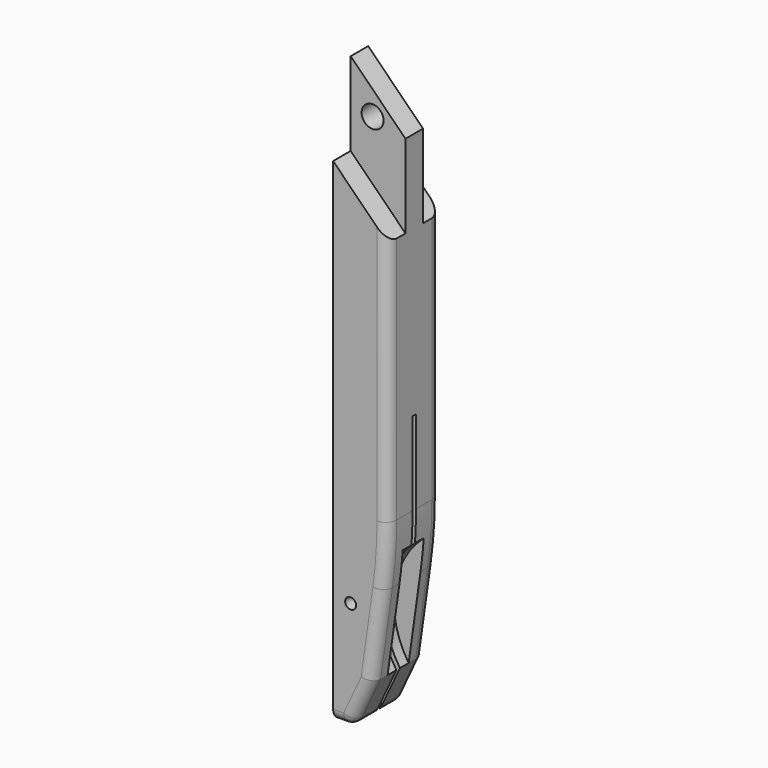
from build123d import *

# Parameters (mm, degrees)
F0_R      = 0.635
F1_DEPTH  = 3.81
F2_R      = 0.635
F3_DEPTH  = 0.254
F5_DEPTH  = 1.524
F7_DEPTH  = 1.524
F9_R      = 1.016
F10_DEPTH = 6.604
F0_R_2    = 1.27
F11_DEPTH = 1.27
F12_R     = 1.27


# Not quite as in the source:
# - two fillets or chamfers of one size are made in one step
# - a pattern or mirror of a feature is missing from the dataset's text; its kind, count and spacing are read off the source's solid


with BuildPart() as f1:
    # F0 (on Front) → F1 (new body)
    with BuildSketch(Plane.XZ):
        with BuildLine():
            Line((6.35, 50.8), (0, 57.15))
            Line((0, 57.15), (0, 0))
            Line((0, 0), (2.032, 0))
            Line((2.032, 0), (4.4819667348, 5.2539706179))
            Line((4.4819667348, 5.2539706179), (5.8556178921, 15.0280064712))
            ThreePointArc((5.8556178921, 15.0280064712), (6.2262537532, 18.5543711338), (6.35, 22.098))
            Line((6.35, 22.098), (6.35, 50.8))
        make_face()
        with Locations((2.032, 12.7)):
            Circle(F0_R, mode=Mode.SUBTRACT)
    extrude(amount=-F1_DEPTH)

    # F1_copies: F1 across plane


with BuildPart() as f1_1:
    add(f1.part)
    add(f1.part.mirror(Plane(origin=(0, 0, 0), x_dir=(0, 0, -1), z_dir=(0, -1, 0))))

    # F2 (on face) → F3 (cut)
    with BuildSketch(Plane.XZ):
        with BuildLine():
            Line((6.35, 31.75), (0, 31.75))
            Line((0, 31.75), (0, 0))
            Line((0, 0), (2.032, 0))
            Line((2.032, 0), (4.4819667348, 5.2539706179))
            Line((4.4819667348, 5.2539706179), (5.8556178921, 15.0280064712))
            ThreePointArc((5.8556178921, 15.0280064712), (6.2262537532, 18.5543711338), (6.35, 22.098))
            Line((6.35, 22.098), (6.35, 31.75))
        make_face()
        with Locations((2.032, 12.7)):
            Circle(F2_R, mode=Mode.SUBTRACT)
    f3 = extrude(amount=-F3_DEPTH, mode=Mode.SUBTRACT)

    # F3_copies: F3 across plane
    add(f3.mirror(Plane(origin=(0, 0, 0), x_dir=(0, 0, -1), z_dir=(0, -1, 0))), mode=Mode.SUBTRACT)

    # F4 (on Front) → F5 (cut, symmetric)
    with BuildSketch(Plane.XZ):
        with BuildLine():
            Line((4.4819667348, 5.2539706179), (4.8144904791, 7.62))
            Line((4.8144904791, 7.62), (5.8556178921, 15.0280064712))
            ThreePointArc((5.8556178921, 15.0280064712), (6.0717122847, 16.787954066), (6.2262537532, 18.5543711338))
            ThreePointArc((6.2262537532, 18.5543711338), (2.8470783684, 12.2329567007), (4.4819667348, 5.2539706179))
        make_face()
        with BuildLine():
            Line((5.8556178921, 15.0280064712), (4.8144904791, 7.62))
            Line((4.8144904791, 7.62), (4.4819667348, 5.2539706179))
            Line((4.4819667348, 5.2539706179), (6.2262537532, 5.0006376953))
            Line((6.2262537532, 5.0006376953), (8.3210639079, 18.5543711338))
            Line((8.3210639079, 18.5543711338), (6.2262537532, 18.5543711338))
            ThreePointArc((6.2262537532, 18.5543711338), (6.0717122847, 16.787954066), (5.8556178921, 15.0280064712))
        make_face()
    extrude(amount=F5_DEPTH, both=True, mode=Mode.SUBTRACT)

    # F4 (on Front) → F7 (cut, symmetric)
    with BuildSketch(Plane.XZ):
        with BuildLine():
            Line((4.4819667348, 5.2539706179), (4.8144904791, 7.62))
            Line((4.8144904791, 7.62), (5.8556178921, 15.0280064712))
            ThreePointArc((5.8556178921, 15.0280064712), (6.0717122847, 16.787954066), (6.2262537532, 18.5543711338))
            ThreePointArc((6.2262537532, 18.5543711338), (2.8470783684, 12.2329567007), (4.4819667348, 5.2539706179))
        make_face()
        with BuildLine():
            Line((5.8556178921, 15.0280064712), (4.8144904791, 7.62))
            Line((4.8144904791, 7.62), (4.4819667348, 5.2539706179))
            Line((4.4819667348, 5.2539706179), (6.2262537532, 5.0006376953))
            Line((6.2262537532, 5.0006376953), (8.3210639079, 18.5543711338))
            Line((8.3210639079, 18.5543711338), (6.2262537532, 18.5543711338))
            ThreePointArc((6.2262537532, 18.5543711338), (6.0717122847, 16.787954066), (5.8556178921, 15.0280064712))
        make_face()
    extrude(amount=F7_DEPTH, both=True, mode=Mode.SUBTRACT)

    # F9 (on face) → F10 (cut)
    with BuildSketch(Plane(origin=(0, 0, 0), x_dir=(0.9747835757, 0, -0.2231523707), z_dir=(0.2231523707, 0, 0.9747835757))):
        with Locations((1.016, 0)):
            Circle(F9_R)
    extrude(amount=F10_DEPTH, mode=Mode.SUBTRACT)

    # F0 (on Front) → F11 (join, symmetric)
    with BuildSketch(Plane.XZ):
        Polygon((0, 66.802), (0, 57.15), (6.35, 50.8), (6.35, 60.452), align=None)
        with Locations((2.54, 61.468)):
            Circle(F0_R_2, mode=Mode.SUBTRACT)
    extrude(amount=F11_DEPTH, both=True)

    # F12 (call 1 of 2: OpenCascade refuses the feature's edges together)
    f12_edges = [f1_1.edges().sort_by_distance(p)[0] for p in [
        (1.016, 3.81, 0),
        (6.35, 3.81, 36.449),
        (6.226254, 3.81, 18.554371),
        (3.256983, 3.81, 2.626985),
        (5.168792, 3.81, 10.140989),
        (2.032, 2.06429, 0),
    ]]
    fillet(f12_edges, radius=F12_R)

    # F12#2 (call 2 of 2)
    f12_2_edges = [f1_1.edges().sort_by_distance(p)[0] for p in [
        (6.35, -3.81, 36.449),
        (1.016, -3.81, 0),
        (3.256983, -3.81, 2.626985),
        (5.168792, -3.81, 10.140989),
        (6.226254, -3.81, 18.554371),
        (2.032, -2.06429, 0),
    ]]
    fillet(f12_2_edges, radius=F12_R)


solid = f1_1.part
